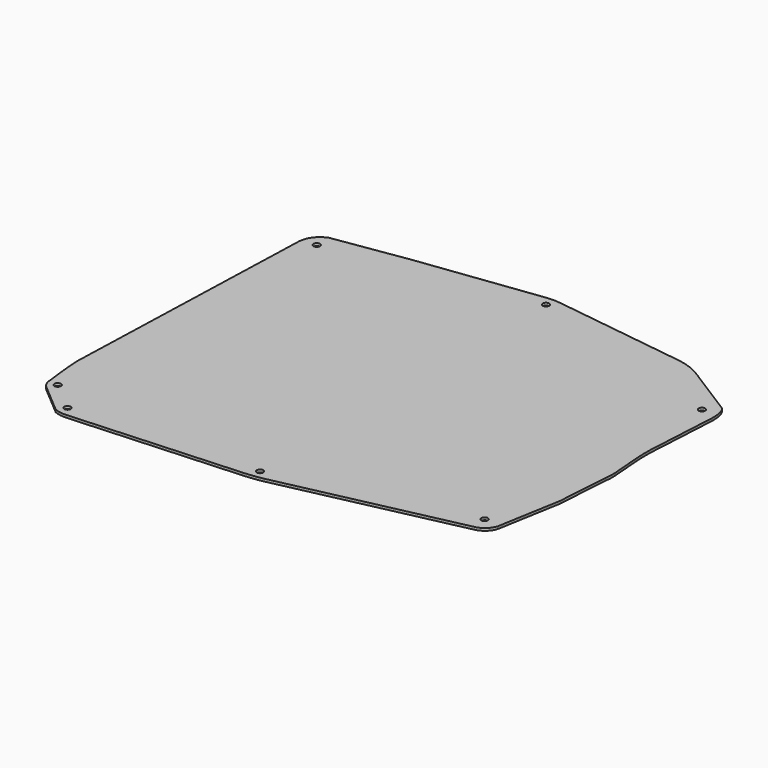
from build123d import *

# Parameters (mm, degrees)
F0_R     = 4.1275
F1_DEPTH = 3.175


# Not quite as in the source:
# - a feature names something its author has since deleted; it is built from what else it names


with BuildPart() as f1:
    # F0 (on Top) → F1 (new body)
    with BuildSketch(Plane.XY):
        with BuildLine():
            Line((81.1441976903, 48.870176137), (118.2163868425, 17.3270926481))
            ThreePointArc((118.2163868425, 17.3270926481), (125.7830950318, 15.1126819317), (133.6548019526, 14.6711869767))
            Line((133.6548019526, 14.6711869767), (347.9302216647, 27.1796528851))
            ThreePointArc((347.9302216647, 27.1796528851), (360.3982548534, 28.3159145983), (372.7658678172, 30.2614458507))
            Line((372.7658678172, 30.2614458507), (601.3625849364, 79.9327344304))
            ThreePointArc((601.3625849364, 79.9327344304), (611.9858366517, 85.4292367374), (618.4030760406, 95.5229998236))
            Line((618.4030760406, 95.5229998236), (632.5431455253, 176.5561104422))
            Line((632.5431455253, 176.5561104422), (636.893926966, 243.6304838067))
            ThreePointArc((636.893926966, 243.6304838067), (637.7262973987, 250.8582634049), (637.6190770743, 258.1330240374))
            Line((637.6190770743, 258.1330240374), (634.718536759, 294.5707376489))
            ThreePointArc((634.718536759, 294.5707376489), (634.0289947151, 313.0653425318), (634.89985466, 331.5522968769))
            Line((634.89985466, 331.5522968769), (639.2500827298, 410.037428213))
            ThreePointArc((639.2500827298, 410.037428213), (638.8544702471, 419.1155099086), (636.6822238963, 427.938741873))
            ThreePointArc((636.6822238963, 427.938741873), (634.7085093964, 431.5717815797), (631.6367376922, 434.3392253523))
            Line((631.6367376922, 434.3392253523), (567.6441777823, 474.7651219969))
            ThreePointArc((567.6441777823, 474.7651219969), (553.0816862682, 482.0654658914), (537.3700250266, 486.3671959048))
            Line((537.3700250266, 486.3671959048), (366.6023005126, 509.5713139182))
            ThreePointArc((366.6023005126, 509.5713139182), (356.5346140159, 510.2066384634), (346.480010855, 509.3899965888))
            Line((346.480010855, 509.3899965888), (192.7528221486, 489.8115695124))
            Line((192.7528221486, 489.8115695124), (99.3925322173, 475.4902721053))
            ThreePointArc((99.3925322173, 475.4902721053), (85.7762927803, 464.7559785435), (80.9017557977, 448.1166899806))
            Line((80.9017557977, 448.1166899806), (69.8140699742, 110.4154438382))
            ThreePointArc((69.8140699742, 110.4154438382), (71.8313111538, 86.8204891023), (74.6482450841, 63.3075982934))
            ThreePointArc((74.6482450841, 63.3075982934), (76.2705931102, 55.3574544062), (81.1441976903, 48.870176137))
        make_face()
        with Locations((125.2569147965, 27.2811080985)):
            Circle(F0_R, mode=Mode.SUBTRACT)
        with Locations((86.803833318, 59.6931402198)):
            Circle(F0_R, mode=Mode.SUBTRACT)
        with Locations((360.0400942892, 40.1343675154)):
            Circle(F0_R, mode=Mode.SUBTRACT)
        with Locations((598.7183749899, 99.1256637739)):
            Circle(F0_R, mode=Mode.SUBTRACT)
        with Locations((99.7337432835, 455.780702147)):
            Circle(F0_R, mode=Mode.SUBTRACT)
        with Locations((357.7462032552, 497.8582725917)):
            Circle(F0_R, mode=Mode.SUBTRACT)
        with Locations((619.9139634468, 418.3134020176)):
            Circle(F0_R, mode=Mode.SUBTRACT)
    extrude(amount=F1_DEPTH)


solid = f1.part
